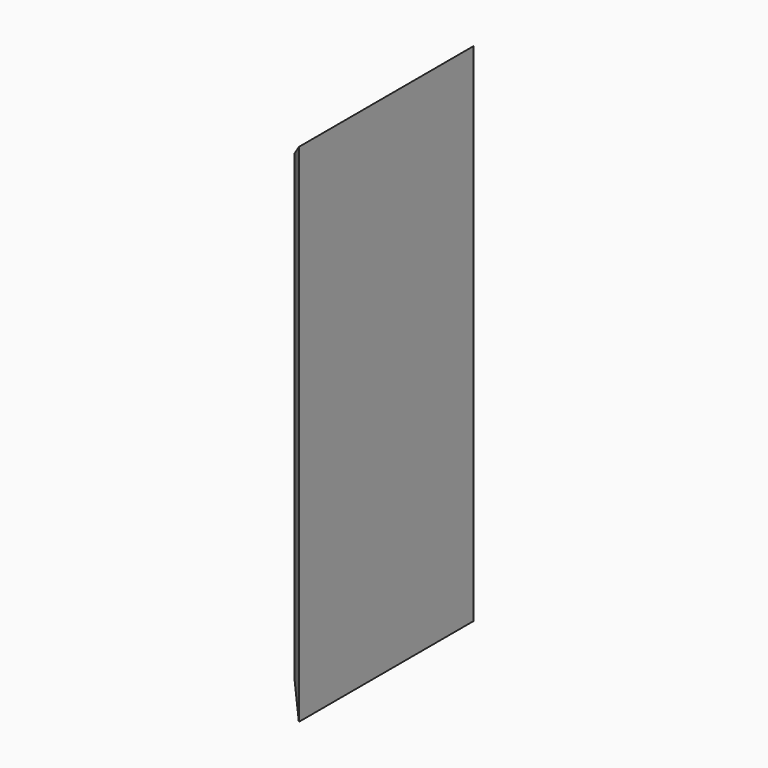
from build123d import *

# Parameters (mm, degrees)
F0_W     = 220
F0_H     = 510
F1_DEPTH = 22
F2_SIZE  = 21.99999


# Not quite as in the source:
# - a fillet or chamfer is up to 0.001 mm smaller than in the source, because OpenCascade refuses the exact size


with BuildPart() as f1:
    # F0 (on Right) → F1 (new body)
    with BuildSketch(Plane.YZ):
        Rectangle(F0_W, F0_H)
    extrude(amount=F1_DEPTH)

    # F2 (size 22 in the source; OpenCascade refuses exactly that, so slightly less here)
    f2_edges = [f1.edges().sort_by_distance(p)[0] for p in [
        (0, 0, 255),
        (0, 110, 0),
        (0, 0, -255),
        (0, -110, 0),
    ]]
    chamfer(f2_edges, length=F2_SIZE)


solid = f1.part
